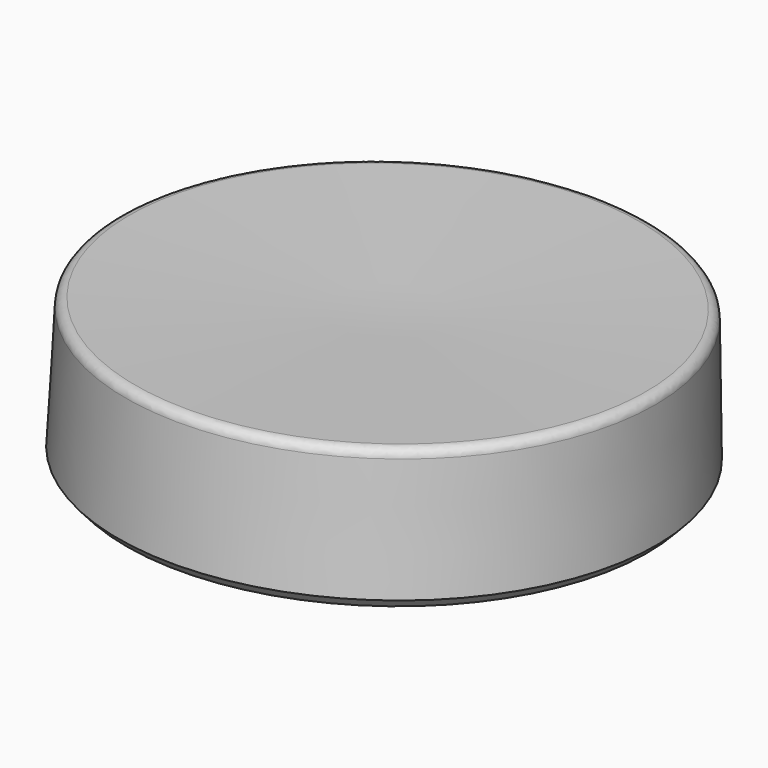
from build123d import *

# Parameters (mm, degrees)
F2_R    = 5.08
F3_SIZE = 5.08


with BuildPart() as f1:
    # F0 (on Right) → F1 (revolve)
    with BuildSketch(Plane.YZ):
        Polygon((-71.8356743455, 79.0152773261), (-74.5772719383, 0), (76.0060697794, 0), (76.0060697794, 79.0152773261), align=None)
    revolve(axis=Axis((0, -73.2064731419, 39.5076386631), (0, -0.0346761903, -0.9993986001)))

    # F2
    f2_edges = [f1.edges().sort_by_distance(p)[0] for p in [
        (0, -219.321877, 89.262288),
    ]]
    fillet(f2_edges, radius=F2_R)

    # F3
    f3_edges = [f1.edges().sort_by_distance(p)[0] for p in [
        (0, -224.798479, 10.437033),
    ]]
    chamfer(f3_edges, length=F3_SIZE)


solid = f1.part
